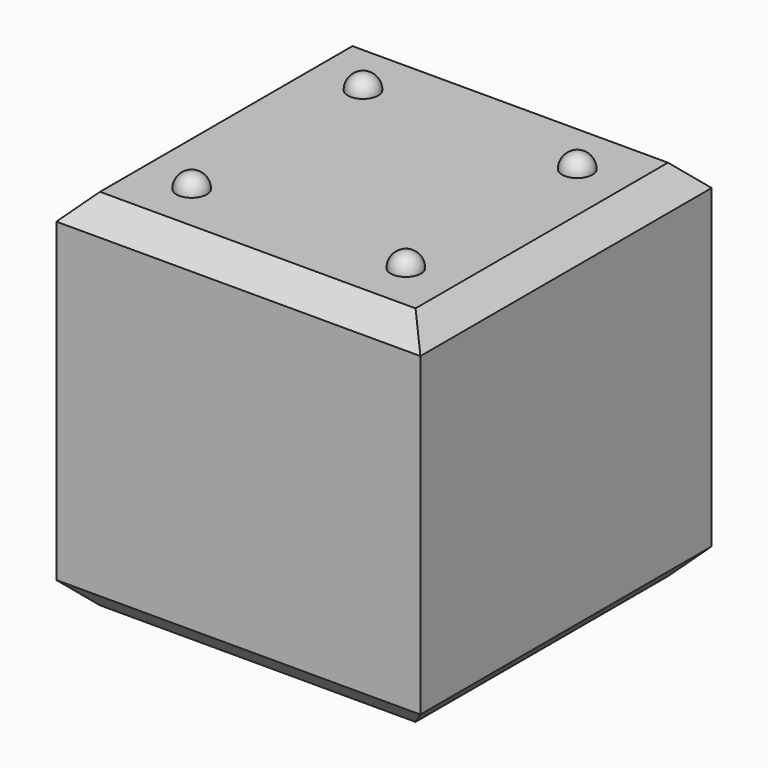
from build123d import *

# Parameters (mm, degrees)
F0_W     = 76.2
F0_H     = 76.2
F1_DEPTH = 76.2
F2_SIZE  = 5.08
F3_R     = 4.953
F4_DEPTH = 25.4
F5_R     = 3.175
F6_DEPTH = 3.175
F7_R     = 3.17499


# Not quite as in the source:
# - a fillet or chamfer is up to 0.001 mm smaller than in the source, because OpenCascade refuses the exact size


with BuildPart() as f1:
    # F0 (on Top) → F1 (new body)
    with BuildSketch(Plane.XY):
        with Locations((-0.4966171047, -21.9681663439)):
            Rectangle(F0_W, F0_H)
    extrude(amount=F1_DEPTH)

    # F2
    f2_edges = [f1.edges().sort_by_distance(p)[0] for p in [
        (-0.496617, -60.068166, 76.2),
        (37.603383, -21.968166, 76.2),
        (-0.496617, 16.131834, 76.2),
        (-38.596617, -21.968166, 76.2),
        (37.603383, -21.968166, 0),
        (-0.496617, -60.068166, 0),
        (-38.596617, -21.968166, 0),
        (-0.496617, 16.131834, 0),
    ]]
    chamfer(f2_edges, length=F2_SIZE)

    # F3 (on face) → F4 (cut)
    with BuildSketch(Plane(origin=(0, 0, 0), x_dir=(1, 0, 0), z_dir=(0, 0, -1))):
        with Locations((0, 21.9681663439)):
            Circle(F3_R)
    extrude(amount=-F4_DEPTH, mode=Mode.SUBTRACT)

    # F5 (on face) → F6 (join)
    with BuildSketch(Plane.XY.offset(76.2)):
        with Locations((-22.4647834486, 0)):
            Circle(F5_R)
        with Locations((22.3648820278, 0)):
            Circle(F5_R)
        with Locations((-22.4647834486, -44.8296654764)):
            Circle(F5_R)
        with Locations((22.3648820278, -44.8296654764)):
            Circle(F5_R)
    extrude(amount=F6_DEPTH)

    # F7 (radius 3.175 in the source; OpenCascade refuses exactly that, so slightly less here)
    f7_edges = [f1.edges().sort_by_distance(p)[0] for p in [
        (-25.639783, -44.829665, 79.375),
        (-25.639783, 0, 79.375),
        (19.189882, 0, 79.375),
        (19.189882, -44.829665, 79.375),
    ]]
    fillet(f7_edges, radius=F7_R)


solid = f1.part
